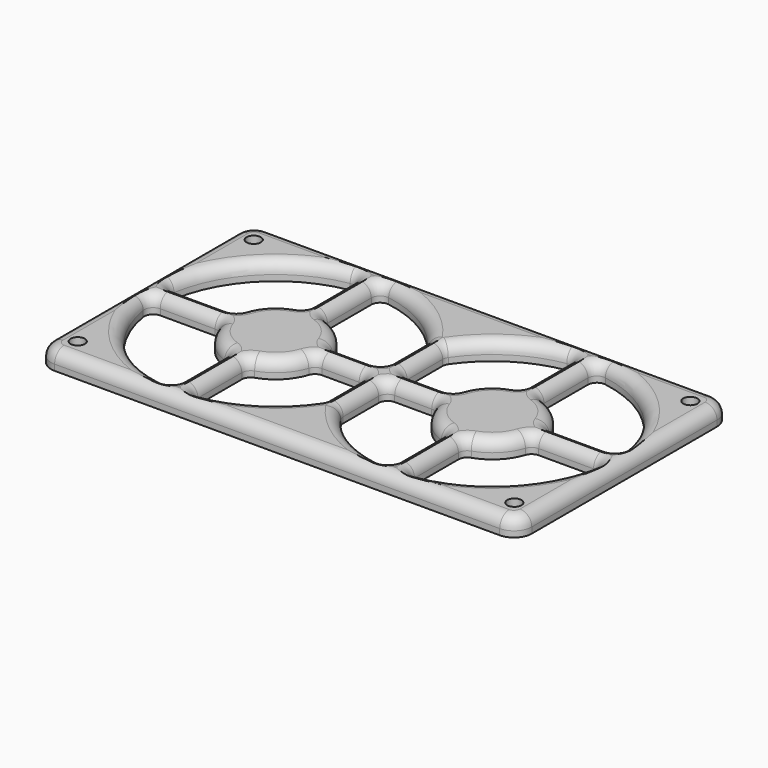
from build123d import *

# Parameters (mm, degrees)
F0_R          = 1.2
F1_DEPTH      = 3
F2_T3_ANGLE   = 71.3351636324
F2_T6_DEPTH   = 9.2412580749
F2_T9_ANGLE   = 53.1830396588
F2_T12_ANGLE  = 53.1830396588
F2_T15_ANGLE  = 46.1876296715
F2_T18_DEPTH  = 7.4731800328
F2_T21_ANGLE  = 53.1830396588
F2_T24_ANGLE  = 53.1830396588
F2_T27_DEPTH  = 39
F2_T30_ANGLE  = 90
F2_T33_ANGLE  = 90
F2_T36_DEPTH  = 75
F2_T39_ANGLE  = 90
F2_T42_DEPTH  = 39
F2_T45_ANGLE  = 90
F2_T48_DEPTH  = 75
F2_T51_ANGLE  = 71.5915198294
F2_T54_ANGLE  = 71.5915198294
F2_T57_DEPTH  = 9.2412580749
F2_T60_ANGLE  = 99.3324181838
F2_T63_ANGLE  = 71.3351636324
F2_T66_ANGLE  = 99.3324181838
F2_T69_DEPTH  = 9.2412580749
F2_T72_ANGLE  = 71.5915198294
F2_T75_ANGLE  = 71.5915198294
F2_T78_DEPTH  = 9.2412580749
F2_T81_ANGLE  = 99.3324181838
F2_T84_ANGLE  = 71.3351636324
F2_T87_ANGLE  = 99.3324181838
F2_T90_DEPTH  = 9.2412580749
F2_T93_ANGLE  = 34.4799521447
F2_T96_ANGLE  = 90
F2_T99_DEPTH  = 6.2361218113
F2_T102_ANGLE = 71.5915198294
F2_T105_ANGLE = 53.1830396588
F2_T108_ANGLE = 71.5915198294
F2_T111_DEPTH = 9.2412580749
F2_T114_ANGLE = 99.3324181838
F2_T117_ANGLE = 46.1876296715
F2_T120_ANGLE = 34.4799521447
F2_T123_ANGLE = 99.3324181838
F2_T126_DEPTH = 9.2412580749
F2_T129_ANGLE = 71.5915198294
F2_T132_ANGLE = 53.1830396588
F2_T135_ANGLE = 71.5915198294
F2_T138_DEPTH = 6.2361218113
F2_T141_ANGLE = 90
F2_T144_DEPTH = 7.4731800328
F2_T147_ANGLE = 71.5915198294
F2_T150_ANGLE = 71.5915198294
F2_T153_DEPTH = 9.2412580749
F2_T156_ANGLE = 99.3324181838
F2_T159_ANGLE = 71.3351636324
F2_T162_ANGLE = 99.3324181838
F2_T165_DEPTH = 9.2412580749
F2_T168_ANGLE = 71.5915198294
F2_T171_ANGLE = 71.5915198294
F2_T174_DEPTH = 9.2412580749
F2_T177_ANGLE = 99.3324181838
F2_T180_ANGLE = 46.1876296715
F2_T183_ANGLE = 34.4799521447
F2_T186_DEPTH = 7.4731800328
F2_T189_ANGLE = 90
F2_T192_DEPTH = 6.2361218113
F2_T195_ANGLE = 99.3324181838
F2_T198_ANGLE = 71.5915198294
F2_T201_ANGLE = 53.1830396588
F2_T204_ANGLE = 71.5915198294
F2_T207_DEPTH = 6.2361218113
F2_T210_ANGLE = 90
F2_T213_DEPTH = 7.4731800328
F2_T216_ANGLE = 34.4799521447
F2_T219_ANGLE = 46.1876296715
F2_T222_ANGLE = 99.3324181838
F2_T225_ANGLE = 99.3324181838
F2_T228_DEPTH = 9.2412580749
F2_T231_ANGLE = 71.5915198294
F2_T234_ANGLE = 53.1830396588
F2_T237_ANGLE = 71.5915198294
F2_T240_DEPTH = 9.2412580749


# Not quite as in the source:
# - a fillet or chamfer that OpenCascade refuses, or shapes differently, is made with other operations: its cross-section is extruded or revolved along the edge and cut away or added


with BuildPart() as f1:
    # F0 (on Top) → F1 (new body)
    with BuildSketch(Plane.XY):
        with BuildLine():
            Line((24.3177403985, -7.9360755384), (-50.6822596015, -7.9360755384))
            ThreePointArc((-50.6822596015, -7.9360755384), (-52.8035799451, -8.8147551948), (-53.6822596015, -10.9360755384))
            Line((-53.6822596015, -10.9360755384), (-53.6822596015, -49.9360755384))
            ThreePointArc((-53.6822596015, -49.9360755384), (-52.8035799451, -52.057395882), (-50.6822596015, -52.9360755384))
            Line((-50.6822596015, -52.9360755384), (24.3177403985, -52.9360755384))
            ThreePointArc((24.3177403985, -52.9360755384), (26.439060742, -52.057395882), (27.3177403985, -49.9360755384))
            Line((27.3177403985, -49.9360755384), (27.3177403985, -10.9360755384))
            ThreePointArc((27.3177403985, -10.9360755384), (26.439060742, -8.8147551948), (24.3177403985, -7.9360755384))
        make_face()
        with Locations((-49.962405785, -48.9713579855)):
            Circle(F0_R, mode=Mode.SUBTRACT)
        with BuildLine():
            ThreePointArc((-34.6703665812, -50.1713579855), (-45.5692589617, -44.5782111621), (-51.162405785, -33.6793187816))
            ThreePointArc((-51.162405785, -33.6793187816), (-50.8256897185, -32.465216348), (-49.6822596015, -31.9360755384))
            Line((-49.6822596015, -31.9360755384), (-40.4410015266, -31.9360755384))
            ThreePointArc((-40.4410015266, -31.9360755384), (-39.5636550488, -32.2194148799), (-39.0177576021, -32.9623913279))
            ThreePointArc((-39.0177576021, -32.9623913279), (-37.0839775875, -36.0929297879), (-33.9534391275, -38.0267098025))
            ThreePointArc((-33.9534391275, -38.0267098025), (-33.2104626795, -38.5726072493), (-32.927123338, -39.4499537271))
            Line((-32.927123338, -39.4499537271), (-32.927123338, -48.6912118019))
            ThreePointArc((-32.927123338, -48.6912118019), (-33.4562641476, -49.8346419189), (-34.6703665812, -50.1713579855))
        make_face(mode=Mode.SUBTRACT)
        with BuildLine():
            ThreePointArc((-28.1838800947, -50.1713579855), (-29.3979825284, -49.8346419189), (-29.927123338, -48.6912118019))
            Line((-29.927123338, -48.6912118019), (-29.927123338, -39.4499537271))
            ThreePointArc((-29.927123338, -39.4499537271), (-29.6437839965, -38.5726072493), (-28.9008075485, -38.0267098025))
            ThreePointArc((-28.9008075485, -38.0267098025), (-25.7702690885, -36.0929297879), (-23.8364890738, -32.9623913279))
            ThreePointArc((-23.8364890738, -32.9623913279), (-23.2905916271, -32.2194148799), (-22.4132451493, -31.9360755384))
            Line((-22.4132451493, -31.9360755384), (-16.177123338, -31.9360755384))
            ThreePointArc((-16.177123338, -31.9360755384), (-15.1164631662, -32.3754153666), (-14.677123338, -33.4360755384))
            Line((-14.677123338, -33.4360755384), (-14.677123338, -40.9092555712))
            ThreePointArc((-14.677123338, -40.9092555712), (-14.7445156231, -41.353817305), (-14.9406368515, -41.7584323306))
            ThreePointArc((-14.9406368515, -41.7584323306), (-20.7028570078, -47.3177256852), (-28.1838800947, -50.1713579855))
        make_face(mode=Mode.SUBTRACT)
        with Locations((23.6081591091, -48.9713579855)):
            Circle(F0_R, mode=Mode.SUBTRACT)
        with BuildLine():
            ThreePointArc((1.8296334188, -50.1713579855), (-5.6513896682, -47.3177256852), (-11.4136098245, -41.7584323306))
            ThreePointArc((-11.4136098245, -41.7584323306), (-11.6097310529, -41.353817305), (-11.677123338, -40.9092555712))
            Line((-11.677123338, -40.9092555712), (-11.677123338, -33.4360755384))
            ThreePointArc((-11.677123338, -33.4360755384), (-11.2377835098, -32.3754153666), (-10.177123338, -31.9360755384))
            Line((-10.177123338, -31.9360755384), (-3.9410015266, -31.9360755384))
            ThreePointArc((-3.9410015266, -31.9360755384), (-3.0636550488, -32.2194148799), (-2.5177576021, -32.9623913279))
            ThreePointArc((-2.5177576021, -32.9623913279), (-0.5839775875, -36.0929297879), (2.5465608725, -38.0267098025))
            ThreePointArc((2.5465608725, -38.0267098025), (3.2895373205, -38.5726072493), (3.572876662, -39.4499537271))
            Line((3.572876662, -39.4499537271), (3.572876662, -48.6912118019))
            ThreePointArc((3.572876662, -48.6912118019), (3.0437358524, -49.8346419189), (1.8296334188, -50.1713579855))
        make_face(mode=Mode.SUBTRACT)
        with BuildLine():
            ThreePointArc((6.572876662, -39.4499537271), (6.8562160035, -38.5726072493), (7.5991924515, -38.0267098025))
            ThreePointArc((7.5991924515, -38.0267098025), (10.7297309115, -36.0929297879), (12.6635109262, -32.9623913279))
            ThreePointArc((12.6635109262, -32.9623913279), (13.2094083729, -32.2194148799), (14.0867548507, -31.9360755384))
            Line((14.0867548507, -31.9360755384), (23.3280129255, -31.9360755384))
            ThreePointArc((23.3280129255, -31.9360755384), (24.4714430425, -32.465216348), (24.8081591091, -33.6793187816))
            ThreePointArc((24.8081591091, -33.6793187816), (19.2150122857, -44.5782111621), (8.3161199053, -50.1713579855))
            ThreePointArc((8.3161199053, -50.1713579855), (7.1020174716, -49.8346419189), (6.572876662, -48.6912118019))
            Line((6.572876662, -48.6912118019), (6.572876662, -39.4499537271))
        make_face(mode=Mode.SUBTRACT)
        with BuildLine():
            ThreePointArc((-34.6703665812, -10.7007930913), (-33.4562641476, -11.0375091579), (-32.927123338, -12.1809392749))
            Line((-32.927123338, -12.1809392749), (-32.927123338, -21.4221973497))
            ThreePointArc((-32.927123338, -21.4221973497), (-33.2104626795, -22.2995438275), (-33.9534391275, -22.8454412743))
            ThreePointArc((-33.9534391275, -22.8454412743), (-37.0839775875, -24.7792212889), (-39.0177576021, -27.9097597489))
            ThreePointArc((-39.0177576021, -27.9097597489), (-39.5636550488, -28.6527361969), (-40.4410015266, -28.9360755384))
            Line((-40.4410015266, -28.9360755384), (-49.6822596015, -28.9360755384))
            ThreePointArc((-49.6822596015, -28.9360755384), (-50.8256897185, -28.4069347288), (-51.162405785, -27.1928322952))
            ThreePointArc((-51.162405785, -27.1928322952), (-45.5692589617, -16.2939399147), (-34.6703665812, -10.7007930913))
        make_face(mode=Mode.SUBTRACT)
        with BuildLine():
            ThreePointArc((-28.9008075485, -22.8454412743), (-29.6437839965, -22.2995438275), (-29.927123338, -21.4221973497))
            Line((-29.927123338, -21.4221973497), (-29.927123338, -12.1809392749))
            ThreePointArc((-29.927123338, -12.1809392749), (-29.3979825284, -11.0375091579), (-28.1838800947, -10.7007930913))
            ThreePointArc((-28.1838800947, -10.7007930913), (-20.7028570078, -13.5544253916), (-14.9406368515, -19.1137187462))
            ThreePointArc((-14.9406368515, -19.1137187462), (-14.7445156231, -19.5183337718), (-14.677123338, -19.9628955056))
            Line((-14.677123338, -19.9628955056), (-14.677123338, -27.4360755384))
            ThreePointArc((-14.677123338, -27.4360755384), (-15.1164631662, -28.4967357102), (-16.177123338, -28.9360755384))
            Line((-16.177123338, -28.9360755384), (-22.4132451493, -28.9360755384))
            ThreePointArc((-22.4132451493, -28.9360755384), (-23.2905916271, -28.6527361969), (-23.8364890738, -27.9097597489))
            ThreePointArc((-23.8364890738, -27.9097597489), (-25.7702690885, -24.7792212889), (-28.9008075485, -22.8454412743))
        make_face(mode=Mode.SUBTRACT)
        with Locations((-49.962405785, -11.9007930913)):
            Circle(F0_R, mode=Mode.SUBTRACT)
        with BuildLine():
            ThreePointArc((1.8296334188, -10.7007930913), (3.0437358524, -11.0375091579), (3.572876662, -12.1809392749))
            Line((3.572876662, -12.1809392749), (3.572876662, -21.4221973497))
            ThreePointArc((3.572876662, -21.4221973497), (3.2895373205, -22.2995438275), (2.5465608725, -22.8454412743))
            ThreePointArc((2.5465608725, -22.8454412743), (-0.5839775875, -24.7792212889), (-2.5177576021, -27.9097597489))
            ThreePointArc((-2.5177576021, -27.9097597489), (-3.0636550488, -28.6527361969), (-3.9410015266, -28.9360755384))
            Line((-3.9410015266, -28.9360755384), (-10.177123338, -28.9360755384))
            ThreePointArc((-10.177123338, -28.9360755384), (-11.2377835098, -28.4967357102), (-11.677123338, -27.4360755384))
            Line((-11.677123338, -27.4360755384), (-11.677123338, -19.9628955056))
            ThreePointArc((-11.677123338, -19.9628955056), (-11.6097310529, -19.5183337718), (-11.4136098245, -19.1137187462))
            ThreePointArc((-11.4136098245, -19.1137187462), (-5.6513896682, -13.5544253916), (1.8296334188, -10.7007930913))
        make_face(mode=Mode.SUBTRACT)
        with BuildLine():
            ThreePointArc((8.3161199053, -10.7007930913), (19.2150122857, -16.2939399147), (24.8081591091, -27.1928322952))
            ThreePointArc((24.8081591091, -27.1928322952), (24.4714430425, -28.4069347288), (23.3280129255, -28.9360755384))
            Line((23.3280129255, -28.9360755384), (14.0867548507, -28.9360755384))
            ThreePointArc((14.0867548507, -28.9360755384), (13.2094083729, -28.6527361969), (12.6635109262, -27.9097597489))
            ThreePointArc((12.6635109262, -27.9097597489), (10.7297309115, -24.7792212889), (7.5991924515, -22.8454412743))
            ThreePointArc((7.5991924515, -22.8454412743), (6.8562160035, -22.2995438275), (6.572876662, -21.4221973497))
            Line((6.572876662, -21.4221973497), (6.572876662, -12.1809392749))
            ThreePointArc((6.572876662, -12.1809392749), (7.1020174716, -11.0375091579), (8.3161199053, -10.7007930913))
        make_face(mode=Mode.SUBTRACT)
        with Locations((23.6081591091, -11.9007930913)):
            Circle(F0_R, mode=Mode.SUBTRACT)
    extrude(amount=F1_DEPTH)

    # F2: fillet of radius 2 on 9 edges, made by hand


with BuildPart() as f2_tool1:
    # F2_s2 → F2_t3 (revolve)
    with BuildSketch(Plane(origin=(9.8097305083, -1.6121047304, 0), x_dir=(0, 0, 1), z_dir=(-0.9867641224, 0.1621621622, 0))):
        with BuildLine():
            ThreePointArc((1, -9.2105987186), (2.4142135624, -8.624812281), (3, -7.2105987186))
            Line((3, -7.2105987186), (3, -9.2105987186))
            Line((3, -9.2105987186), (1, -9.2105987186))
        make_face()
    revolve(axis=Axis((5.072876662, -30.4360755384, 3), (0, 0, -1)), revolution_arc=F2_T3_ANGLE)


with BuildPart() as f2_tool4:
    # F2_s5 → F2_t6 (new body)
    with BuildSketch(Plane.XZ.offset(12.1809392749)):
        with BuildLine():
            ThreePointArc((3.572876662, 1), (4.1586630996, 2.4142135624), (5.572876662, 3))
            Line((5.572876662, 3), (3.572876662, 3))
            Line((3.572876662, 3), (3.572876662, 1))
        make_face()
    extrude(amount=F2_T6_DEPTH)


with BuildPart() as f2_tool7:
    # F2_s8 → F2_t9 (revolve)
    with BuildSketch(Plane(origin=(9.6254528786, -28.920886586, 0), x_dir=(0, 0, 1), z_dir=(-0.3157894737, 0.948829283, 0))):
        with BuildLine():
            ThreePointArc((1, -12.7980983492), (2.4142135624, -12.2123119116), (3, -10.7980983492))
            Line((3, -10.7980983492), (3, -12.7980983492))
            Line((3, -12.7980983492), (1, -12.7980983492))
        make_face()
    revolve(axis=Axis((5.072876662, -30.4360755384, 3), (0, 0, 1)), revolution_arc=F2_T9_ANGLE)


with BuildPart() as f2_tool10:
    # F2_s11 → F2_t12 (revolve)
    with BuildSketch(Plane(origin=(-4.5525762165, -1.5151889524, 0), x_dir=(0, 0, 1), z_dir=(-0.948829283, -0.3157894737, 0))):
        with BuildLine():
            ThreePointArc((1, -38.4806007821), (2.4142135624, -37.8948143445), (3, -36.4806007821))
            Line((3, -36.4806007821), (3, -38.4806007821))
            Line((3, -38.4806007821), (1, -38.4806007821))
        make_face()
    revolve(axis=Axis((5.072876662, -30.4360755384, 3), (0, 0, 1)), revolution_arc=F2_T12_ANGLE)


with BuildPart() as f2_tool13:
    # F2_s14 → F2_t15 (revolve)
    with BuildSketch(Plane(origin=(-24.2755023956, -35.3475649585, 0), x_dir=(0, 0, 1), z_dir=(0.5661178396, 0.8243243243, 0))):
        with BuildLine():
            ThreePointArc((1, 11.324263119), (2.4142135624, 11.9100495567), (3, 13.324263119))
            Line((3, 13.324263119), (3, 11.324263119))
            Line((3, 11.324263119), (1, 11.324263119))
        make_face()
    revolve(axis=Axis((-31.427123338, -30.4360755384, 3), (0, 0, -1)), revolution_arc=F2_T15_ANGLE)


with BuildPart() as f2_tool16:
    # F2_s17 → F2_t18 (new body)
    with BuildSketch(Plane.XZ.offset(19.9628955056)):
        with BuildLine():
            ThreePointArc((-14.677123338, 1), (-14.0913369004, 2.4142135624), (-12.677123338, 3))
            Line((-12.677123338, 3), (-14.677123338, 3))
            Line((-14.677123338, 3), (-14.677123338, 1))
        make_face()
    extrude(amount=F2_T18_DEPTH)


with BuildPart() as f2_tool19:
    # F2_s20 → F2_t21 (revolve)
    with BuildSketch(Plane(origin=(-37.4126870199, -12.4516948987, 0), x_dir=(0, 0, 1), z_dir=(0.948829283, 0.3157894737, 0))):
        with BuildLine():
            ThreePointArc((1, 10.9542849926), (2.4142135624, 11.5400714303), (3, 12.9542849926))
            Line((3, 12.9542849926), (3, 10.9542849926))
            Line((3, 10.9542849926), (1, 10.9542849926))
        make_face()
    revolve(axis=Axis((-31.427123338, -30.4360755384, 3), (0, 0, 1)), revolution_arc=F2_T21_ANGLE)


with BuildPart() as f2_tool22:
    # F2_s23 → F2_t24 (revolve)
    with BuildSketch(Plane(origin=(5.9855636819, -17.9843806397, 0), x_dir=(0, 0, 1), z_dir=(-0.3157894737, 0.948829283, 0))):
        with BuildLine():
            ThreePointArc((1, -47.4303671793), (2.4142135624, -46.8445807417), (3, -45.4303671793))
            Line((3, -45.4303671793), (3, -47.4303671793))
            Line((3, -47.4303671793), (1, -47.4303671793))
        make_face()
    revolve(axis=Axis((-31.427123338, -30.4360755384, 3), (0, 0, 1)), revolution_arc=F2_T24_ANGLE)


with BuildPart() as f2_tool25:
    # F2_s26 → F2_t27 (new body)
    with BuildSketch(Plane.XZ.offset(10.9360755384)):
        with BuildLine():
            ThreePointArc((-53.6822596015, 1), (-53.0964731639, 2.4142135624), (-51.6822596015, 3))
            Line((-51.6822596015, 3), (-53.6822596015, 3))
            Line((-53.6822596015, 3), (-53.6822596015, 1))
        make_face()
    extrude(amount=F2_T27_DEPTH)


with BuildPart() as f2_tool28:
    # F2_s29 → F2_t30 (revolve)
    with BuildSketch(Plane.YZ.offset(-50.6822596015)):
        with BuildLine():
            ThreePointArc((-7.9360755384, 1), (-8.521861976, 2.4142135624), (-9.9360755384, 3))
            Line((-9.9360755384, 3), (-7.9360755384, 3))
            Line((-7.9360755384, 3), (-7.9360755384, 1))
        make_face()
    revolve(axis=Axis((-50.6822596015, -10.9360755384, 3), (0, 0, 1)), revolution_arc=F2_T30_ANGLE)


with BuildPart() as f2_tool31:
    # F2_s32 → F2_t33 (revolve)
    with BuildSketch(Plane.XZ.offset(49.9360755384)):
        with BuildLine():
            ThreePointArc((-53.6822596015, 1), (-53.0964731639, 2.4142135624), (-51.6822596015, 3))
            Line((-51.6822596015, 3), (-53.6822596015, 3))
            Line((-53.6822596015, 3), (-53.6822596015, 1))
        make_face()
    revolve(axis=Axis((-50.6822596015, -49.9360755384, 3), (0, 0, 1)), revolution_arc=F2_T33_ANGLE)


with BuildPart() as f2_tool34:
    # F2_s35 → F2_t36 (new body)
    with BuildSketch(Plane.YZ.offset(-50.6822596015)):
        with BuildLine():
            ThreePointArc((-52.9360755384, 1), (-52.3502891008, 2.4142135624), (-50.9360755384, 3))
            Line((-50.9360755384, 3), (-52.9360755384, 3))
            Line((-52.9360755384, 3), (-52.9360755384, 1))
        make_face()
    extrude(amount=F2_T36_DEPTH)


with BuildPart() as f2_tool37:
    # F2_s38 → F2_t39 (revolve)
    with BuildSketch(Plane.YZ.offset(24.3177403985)):
        with BuildLine():
            ThreePointArc((-52.9360755384, 1), (-52.3502891008, 2.4142135624), (-50.9360755384, 3))
            Line((-50.9360755384, 3), (-52.9360755384, 3))
            Line((-52.9360755384, 3), (-52.9360755384, 1))
        make_face()
    revolve(axis=Axis((24.3177403985, -49.9360755384, 3), (0, 0, 1)), revolution_arc=F2_T39_ANGLE)


with BuildPart() as f2_tool40:
    # F2_s41 → F2_t42 (new body)
    with BuildSketch(Plane.XZ.offset(49.9360755384)):
        with BuildLine():
            ThreePointArc((27.3177403985, 1), (26.7319539609, 2.4142135624), (25.3177403985, 3))
            Line((25.3177403985, 3), (27.3177403985, 3))
            Line((27.3177403985, 3), (27.3177403985, 1))
        make_face()
    extrude(amount=-F2_T42_DEPTH)


with BuildPart() as f2_tool43:
    # F2_s44 → F2_t45 (revolve)
    with BuildSketch(Plane.XZ.offset(10.9360755384)):
        with BuildLine():
            ThreePointArc((27.3177403985, 1), (26.7319539609, 2.4142135624), (25.3177403985, 3))
            Line((25.3177403985, 3), (27.3177403985, 3))
            Line((27.3177403985, 3), (27.3177403985, 1))
        make_face()
    revolve(axis=Axis((24.3177403985, -10.9360755384, 3), (0, 0, 1)), revolution_arc=F2_T45_ANGLE)


with BuildPart() as f2_tool46:
    # F2_s47 → F2_t48 (new body)
    with BuildSketch(Plane.YZ.offset(24.3177403985)):
        with BuildLine():
            ThreePointArc((-7.9360755384, 1), (-8.521861976, 2.4142135624), (-9.9360755384, 3))
            Line((-9.9360755384, 3), (-7.9360755384, 3))
            Line((-7.9360755384, 3), (-7.9360755384, 1))
        make_face()
    extrude(amount=-F2_T48_DEPTH)


with BuildPart() as f2_tool49:
    # F2_s50 → F2_t51 (revolve)
    with BuildSketch(Plane.YZ.offset(-40.4410015266)):
        with BuildLine():
            ThreePointArc((-31.9360755384, 1), (-31.3502891008, 2.4142135624), (-29.9360755384, 3))
            Line((-29.9360755384, 3), (-31.9360755384, 3))
            Line((-31.9360755384, 3), (-31.9360755384, 1))
        make_face()
    revolve(axis=Axis((-40.4410015266, -33.4360755384, 3), (0, 0, -1)), revolution_arc=F2_T51_ANGLE)


with BuildPart() as f2_tool52:
    # F2_s53 → F2_t54 (revolve)
    with BuildSketch(Plane(origin=(-19.1735461372, 6.3813418828, 0), x_dir=(0, 0, 1), z_dir=(-0.948829283, 0.3157894737, 0))):
        with BuildLine():
            ThreePointArc((1, -46.8029944693), (2.4142135624, -46.2172080316), (3, -44.8029944693))
            Line((3, -44.8029944693), (3, -46.8029944693))
            Line((3, -46.8029944693), (1, -46.8029944693))
        make_face()
    revolve(axis=Axis((-34.427123338, -39.4499537271, 3), (0, 0, -1)), revolution_arc=F2_T54_ANGLE)


with BuildPart() as f2_tool55:
    # F2_s56 → F2_t57 (new body)
    with BuildSketch(Plane.XZ.offset(39.4499537271)):
        with BuildLine():
            ThreePointArc((-32.927123338, 1), (-32.3413369004, 2.4142135624), (-30.927123338, 3))
            Line((-30.927123338, 3), (-32.927123338, 3))
            Line((-32.927123338, 3), (-32.927123338, 1))
        make_face()
    extrude(amount=F2_T57_DEPTH)


with BuildPart() as f2_tool58:
    # F2_s59 → F2_t60 (revolve)
    with BuildSketch(Plane.XZ.offset(48.6912118019)):
        with BuildLine():
            ThreePointArc((-32.927123338, 1), (-32.3413369004, 2.4142135624), (-30.927123338, 3))
            Line((-30.927123338, 3), (-32.927123338, 3))
            Line((-32.927123338, 3), (-32.927123338, 1))
        make_face()
    revolve(axis=Axis((-34.427123338, -48.6912118019, 3), (0, 0, -1)), revolution_arc=F2_T60_ANGLE)


with BuildPart() as f2_tool61:
    # F2_s62 → F2_t63 (revolve)
    with BuildSketch(Plane(origin=(-25.7304448022, 4.2284721019, 0), x_dir=(0, 0, 1), z_dir=(0.9867641224, -0.1621621622, 0))):
        with BuildLine():
            ThreePointArc((1, 55.1295176375), (2.4142135624, 55.7153040752), (3, 57.1295176375))
            Line((3, 57.1295176375), (3, 55.1295176375))
            Line((3, 55.1295176375), (1, 55.1295176375))
        make_face()
    revolve(axis=Axis((-31.427123338, -30.4360755384, 3), (0, 0, -1)), revolution_arc=F2_T63_ANGLE)


with BuildPart() as f2_tool64:
    # F2_s65 → F2_t66 (revolve)
    with BuildSketch(Plane(origin=(4.0438276371, -24.6068748472, 0), x_dir=(0, 0, 1), z_dir=(0.1621621622, -0.9867641224, 0))):
        with BuildLine():
            ThreePointArc((1, 55.9467375957), (2.4142135624, 56.5325240333), (3, 57.9467375957))
            Line((3, 57.9467375957), (3, 55.9467375957))
            Line((3, 55.9467375957), (1, 55.9467375957))
        make_face()
    revolve(axis=Axis((-49.6822596015, -33.4360755384, 3), (0, 0, -1)), revolution_arc=F2_T66_ANGLE)


with BuildPart() as f2_tool67:
    # F2_s68 → F2_t69 (new body)
    with BuildSketch(Plane.YZ.offset(-49.6822596015)):
        with BuildLine():
            ThreePointArc((-31.9360755384, 1), (-31.3502891008, 2.4142135624), (-29.9360755384, 3))
            Line((-29.9360755384, 3), (-31.9360755384, 3))
            Line((-31.9360755384, 3), (-31.9360755384, 1))
        make_face()
    extrude(amount=F2_T69_DEPTH)


with BuildPart() as f2_tool70:
    # F2_s71 → F2_t72 (revolve)
    with BuildSketch(Plane.XZ.offset(21.4221973497)):
        with BuildLine():
            ThreePointArc((-32.927123338, 1), (-32.3413369004, 2.4142135624), (-30.927123338, 3))
            Line((-30.927123338, 3), (-32.927123338, 3))
            Line((-32.927123338, 3), (-32.927123338, 1))
        make_face()
    revolve(axis=Axis((-34.427123338, -21.4221973497, 3), (0, 0, -1)), revolution_arc=F2_T72_ANGLE)


with BuildPart() as f2_tool73:
    # F2_s74 → F2_t75 (revolve)
    with BuildSketch(Plane(origin=(-12.2535772008, -36.8174174212, 0), x_dir=(0, 0, 1), z_dir=(0.3157894737, 0.948829283, 0))):
        with BuildLine():
            ThreePointArc((1, -28.2075826288), (2.4142135624, -27.6217961912), (3, -26.2075826288))
            Line((3, -26.2075826288), (3, -28.2075826288))
            Line((3, -28.2075826288), (1, -28.2075826288))
        make_face()
    revolve(axis=Axis((-40.4410015266, -27.4360755384, 3), (0, 0, -1)), revolution_arc=F2_T75_ANGLE)


with BuildPart() as f2_tool76:
    # F2_s77 → F2_t78 (new body)
    with BuildSketch(Plane.YZ.offset(-40.4410015266)):
        with BuildLine():
            ThreePointArc((-28.9360755384, 1), (-29.521861976, 2.4142135624), (-30.9360755384, 3))
            Line((-30.9360755384, 3), (-28.9360755384, 3))
            Line((-28.9360755384, 3), (-28.9360755384, 1))
        make_face()
    extrude(amount=-F2_T78_DEPTH)


with BuildPart() as f2_tool79:
    # F2_s80 → F2_t81 (revolve)
    with BuildSketch(Plane.YZ.offset(-49.6822596015)):
        with BuildLine():
            ThreePointArc((-28.9360755384, 1), (-29.521861976, 2.4142135624), (-30.9360755384, 3))
            Line((-30.9360755384, 3), (-28.9360755384, 3))
            Line((-28.9360755384, 3), (-28.9360755384, 1))
        make_face()
    revolve(axis=Axis((-49.6822596015, -27.4360755384, 3), (0, 0, -1)), revolution_arc=F2_T81_ANGLE)


with BuildPart() as f2_tool82:
    # F2_s83 → F2_t84 (revolve)
    with BuildSketch(Plane(origin=(-5.6966785358, -34.6645476403, 0), x_dir=(0, 0, 1), z_dir=(-0.1621621622, -0.9867641224, 0))):
        with BuildLine():
            ThreePointArc((1, 46.0755779616), (2.4142135624, 46.6613643993), (3, 48.0755779616))
            Line((3, 48.0755779616), (3, 46.0755779616))
            Line((3, 46.0755779616), (1, 46.0755779616))
        make_face()
    revolve(axis=Axis((-31.427123338, -30.4360755384, 3), (0, 0, -1)), revolution_arc=F2_T84_ANGLE)


with BuildPart() as f2_tool85:
    # F2_s86 → F2_t87 (revolve)
    with BuildSketch(Plane(origin=(-35.4709509751, -5.8292006912, 0), x_dir=(0, 0, 1), z_dir=(-0.9867641224, -0.1621621622, 0))):
        with BuildLine():
            ThreePointArc((1, -4.9369370955), (2.4142135624, -4.3511506579), (3, -2.9369370955))
            Line((3, -2.9369370955), (3, -4.9369370955))
            Line((3, -4.9369370955), (1, -4.9369370955))
        make_face()
    revolve(axis=Axis((-34.427123338, -12.1809392749, 3), (0, 0, -1)), revolution_arc=F2_T87_ANGLE)


with BuildPart() as f2_tool88:
    # F2_s89 → F2_t90 (new body)
    with BuildSketch(Plane.XZ.offset(12.1809392749)):
        with BuildLine():
            ThreePointArc((-32.927123338, 1), (-32.3413369004, 2.4142135624), (-30.927123338, 3))
            Line((-30.927123338, 3), (-32.927123338, 3))
            Line((-32.927123338, 3), (-32.927123338, 1))
        make_face()
    extrude(amount=F2_T90_DEPTH)


with BuildPart() as f2_tool91:
    # F2_s92 → F2_t93 (revolve)
    with BuildSketch(Plane(origin=(4.1313820675, -6.0157064361, 0), x_dir=(0, 0, 1), z_dir=(-0.5661178396, 0.8243243243, 0))):
        with BuildLine():
            ThreePointArc((1, -23.1365475411), (2.4142135624, -22.5507611035), (3, -21.1365475411))
            Line((3, -21.1365475411), (3, -23.1365475411))
            Line((3, -23.1365475411), (1, -23.1365475411))
        make_face()
    revolve(axis=Axis((-16.177123338, -19.9628955056, 3), (0, 0, -1)), revolution_arc=F2_T93_ANGLE)


with BuildPart() as f2_tool94:
    # F2_s95 → F2_t96 (revolve)
    with BuildSketch(Plane.XZ.offset(27.4360755384)):
        with BuildLine():
            ThreePointArc((-14.677123338, 1), (-14.0913369004, 2.4142135624), (-12.677123338, 3))
            Line((-12.677123338, 3), (-14.677123338, 3))
            Line((-14.677123338, 3), (-14.677123338, 1))
        make_face()
    revolve(axis=Axis((-16.177123338, -27.4360755384, 3), (0, 0, -1)), revolution_arc=F2_T96_ANGLE)


with BuildPart() as f2_tool97:
    # F2_s98 → F2_t99 (new body)
    with BuildSketch(Plane.YZ.offset(-16.177123338)):
        with BuildLine():
            ThreePointArc((-28.9360755384, 1), (-29.521861976, 2.4142135624), (-30.9360755384, 3))
            Line((-30.9360755384, 3), (-28.9360755384, 3))
            Line((-28.9360755384, 3), (-28.9360755384, 1))
        make_face()
    extrude(amount=-F2_T99_DEPTH)


with BuildPart() as f2_tool100:
    # F2_s101 → F2_t102 (revolve)
    with BuildSketch(Plane.YZ.offset(-22.4132451493)):
        with BuildLine():
            ThreePointArc((-28.9360755384, 1), (-29.521861976, 2.4142135624), (-30.9360755384, 3))
            Line((-30.9360755384, 3), (-28.9360755384, 3))
            Line((-28.9360755384, 3), (-28.9360755384, 1))
        make_face()
    revolve(axis=Axis((-22.4132451493, -27.4360755384, 3), (0, 0, -1)), revolution_arc=F2_T102_ANGLE)


with BuildPart() as f2_tool103:
    # F2_s104 → F2_t105 (revolve)
    with BuildSketch(Plane(origin=(5.9855636819, -17.9843806397, 0), x_dir=(0, 0, 1), z_dir=(0.3157894737, -0.948829283, 0))):
        with BuildLine():
            ThreePointArc((1, 31.4303671793), (2.4142135624, 32.016153617), (3, 33.4303671793))
            Line((3, 33.4303671793), (3, 31.4303671793))
            Line((3, 31.4303671793), (1, 31.4303671793))
        make_face()
    revolve(axis=Axis((-31.427123338, -30.4360755384, 3), (0, 0, 1)), revolution_arc=F2_T105_ANGLE)


with BuildPart() as f2_tool106:
    # F2_s107 → F2_t108 (revolve)
    with BuildSketch(Plane(origin=(-19.1735461372, 6.3813418828, 0), x_dir=(0, 0, 1), z_dir=(0.948829283, -0.3157894737, 0))):
        with BuildLine():
            ThreePointArc((1, 30.8029944693), (2.4142135624, 31.3887809069), (3, 32.8029944693))
            Line((3, 32.8029944693), (3, 30.8029944693))
            Line((3, 30.8029944693), (1, 30.8029944693))
        make_face()
    revolve(axis=Axis((-28.427123338, -21.4221973497, 3), (0, 0, -1)), revolution_arc=F2_T108_ANGLE)


with BuildPart() as f2_tool109:
    # F2_s110 → F2_t111 (new body)
    with BuildSketch(Plane.XZ.offset(21.4221973497)):
        with BuildLine():
            ThreePointArc((-29.927123338, 1), (-30.5129097756, 2.4142135624), (-31.927123338, 3))
            Line((-31.927123338, 3), (-29.927123338, 3))
            Line((-29.927123338, 3), (-29.927123338, 1))
        make_face()
    extrude(amount=-F2_T111_DEPTH)


with BuildPart() as f2_tool112:
    # F2_s113 → F2_t114 (revolve)
    with BuildSketch(Plane.XZ.offset(12.1809392749)):
        with BuildLine():
            ThreePointArc((-29.927123338, 1), (-30.5129097756, 2.4142135624), (-31.927123338, 3))
            Line((-31.927123338, 3), (-29.927123338, 3))
            Line((-29.927123338, 3), (-29.927123338, 1))
        make_face()
    revolve(axis=Axis((-28.427123338, -12.1809392749, 3), (0, 0, -1)), revolution_arc=F2_T114_ANGLE)


with BuildPart() as f2_tool115:
    # F2_s116 → F2_t117 (revolve)
    with BuildSketch(Plane(origin=(-25.7304448022, 4.2284721019, 0), x_dir=(0, 0, 1), z_dir=(-0.9867641224, 0.1621621622, 0))):
        with BuildLine():
            ThreePointArc((1, -15.1295176375), (2.4142135624, -14.5437311999), (3, -13.1295176375))
            Line((3, -13.1295176375), (3, -15.1295176375))
            Line((3, -15.1295176375), (1, -15.1295176375))
        make_face()
    revolve(axis=Axis((-31.427123338, -30.4360755384, 3), (0, 0, -1)), revolution_arc=F2_T117_ANGLE)


with BuildPart() as f2_tool118:
    # F2_s119 → F2_t120 (revolve)
    with BuildSketch(Plane.XZ.offset(40.9092555712)):
        with BuildLine():
            ThreePointArc((-14.677123338, 1), (-14.0913369004, 2.4142135624), (-12.677123338, 3))
            Line((-12.677123338, 3), (-14.677123338, 3))
            Line((-14.677123338, 3), (-14.677123338, 1))
        make_face()
    revolve(axis=Axis((-16.177123338, -40.9092555712, 3), (0, 0, -1)), revolution_arc=F2_T120_ANGLE)


with BuildPart() as f2_tool121:
    # F2_s122 → F2_t123 (revolve)
    with BuildSketch(Plane(origin=(-35.4709509751, -5.8292006912, 0), x_dir=(0, 0, 1), z_dir=(0.9867641224, 0.1621621622, 0))):
        with BuildLine():
            ThreePointArc((1, 44.9369370955), (2.4142135624, 45.5227235331), (3, 46.9369370955))
            Line((3, 46.9369370955), (3, 44.9369370955))
            Line((3, 44.9369370955), (1, 44.9369370955))
        make_face()
    revolve(axis=Axis((-28.427123338, -48.6912118019, 3), (0, 0, -1)), revolution_arc=F2_T123_ANGLE)


with BuildPart() as f2_tool124:
    # F2_s125 → F2_t126 (new body)
    with BuildSketch(Plane.XZ.offset(48.6912118019)):
        with BuildLine():
            ThreePointArc((-29.927123338, 1), (-30.5129097756, 2.4142135624), (-31.927123338, 3))
            Line((-31.927123338, 3), (-29.927123338, 3))
            Line((-29.927123338, 3), (-29.927123338, 1))
        make_face()
    extrude(amount=-F2_T126_DEPTH)


with BuildPart() as f2_tool127:
    # F2_s128 → F2_t129 (revolve)
    with BuildSketch(Plane.XZ.offset(39.4499537271)):
        with BuildLine():
            ThreePointArc((-29.927123338, 1), (-30.5129097756, 2.4142135624), (-31.927123338, 3))
            Line((-31.927123338, 3), (-29.927123338, 3))
            Line((-29.927123338, 3), (-29.927123338, 1))
        make_face()
    revolve(axis=Axis((-28.427123338, -39.4499537271, 3), (0, 0, -1)), revolution_arc=F2_T129_ANGLE)


with BuildPart() as f2_tool130:
    # F2_s131 → F2_t132 (revolve)
    with BuildSketch(Plane(origin=(-37.4126870199, -12.4516948987, 0), x_dir=(0, 0, 1), z_dir=(-0.948829283, -0.3157894737, 0))):
        with BuildLine():
            ThreePointArc((1, -26.9542849926), (2.4142135624, -26.368498555), (3, -24.9542849926))
            Line((3, -24.9542849926), (3, -26.9542849926))
            Line((3, -26.9542849926), (1, -26.9542849926))
        make_face()
    revolve(axis=Axis((-31.427123338, -30.4360755384, 3), (0, 0, 1)), revolution_arc=F2_T132_ANGLE)


with BuildPart() as f2_tool133:
    # F2_s134 → F2_t135 (revolve)
    with BuildSketch(Plane(origin=(-12.2535772008, -36.8174174212, 0), x_dir=(0, 0, 1), z_dir=(-0.3157894737, -0.948829283, 0))):
        with BuildLine():
            ThreePointArc((1, 12.2075826288), (2.4142135624, 12.7933690664), (3, 14.2075826288))
            Line((3, 14.2075826288), (3, 12.2075826288))
            Line((3, 12.2075826288), (1, 12.2075826288))
        make_face()
    revolve(axis=Axis((-22.4132451493, -33.4360755384, 3), (0, 0, -1)), revolution_arc=F2_T135_ANGLE)


with BuildPart() as f2_tool136:
    # F2_s137 → F2_t138 (new body)
    with BuildSketch(Plane.YZ.offset(-22.4132451493)):
        with BuildLine():
            ThreePointArc((-31.9360755384, 1), (-31.3502891008, 2.4142135624), (-29.9360755384, 3))
            Line((-29.9360755384, 3), (-31.9360755384, 3))
            Line((-31.9360755384, 3), (-31.9360755384, 1))
        make_face()
    extrude(amount=F2_T138_DEPTH)


with BuildPart() as f2_tool139:
    # F2_s140 → F2_t141 (revolve)
    with BuildSketch(Plane.YZ.offset(-16.177123338)):
        with BuildLine():
            ThreePointArc((-31.9360755384, 1), (-31.3502891008, 2.4142135624), (-29.9360755384, 3))
            Line((-29.9360755384, 3), (-31.9360755384, 3))
            Line((-31.9360755384, 3), (-31.9360755384, 1))
        make_face()
    revolve(axis=Axis((-16.177123338, -33.4360755384, 3), (0, 0, -1)), revolution_arc=F2_T141_ANGLE)


with BuildPart() as f2_tool142:
    # F2_s143 → F2_t144 (new body)
    with BuildSketch(Plane.XZ.offset(33.4360755384)):
        with BuildLine():
            ThreePointArc((-14.677123338, 1), (-14.0913369004, 2.4142135624), (-12.677123338, 3))
            Line((-12.677123338, 3), (-14.677123338, 3))
            Line((-14.677123338, 3), (-14.677123338, 1))
        make_face()
    extrude(amount=F2_T144_DEPTH)


with BuildPart() as f2_tool145:
    # F2_s146 → F2_t147 (revolve)
    with BuildSketch(Plane.XZ.offset(39.4499537271)):
        with BuildLine():
            ThreePointArc((6.572876662, 1), (5.9870902244, 2.4142135624), (4.572876662, 3))
            Line((4.572876662, 3), (6.572876662, 3))
            Line((6.572876662, 3), (6.572876662, 1))
        make_face()
    revolve(axis=Axis((8.072876662, -39.4499537271, 3), (0, 0, -1)), revolution_arc=F2_T147_ANGLE)


with BuildPart() as f2_tool148:
    # F2_s149 → F2_t150 (revolve)
    with BuildSketch(Plane(origin=(-8.6136880041, -25.8809114748, 0), x_dir=(0, 0, 1), z_dir=(-0.3157894737, -0.948829283, 0))):
        with BuildLine():
            ThreePointArc((1, -22.4246862013), (2.4142135624, -21.8388997637), (3, -20.4246862013))
            Line((3, -20.4246862013), (3, -22.4246862013))
            Line((3, -22.4246862013), (1, -22.4246862013))
        make_face()
    revolve(axis=Axis((14.0867548507, -33.4360755384, 3), (0, 0, -1)), revolution_arc=F2_T150_ANGLE)


with BuildPart() as f2_tool151:
    # F2_s152 → F2_t153 (new body)
    with BuildSketch(Plane.YZ.offset(14.0867548507)):
        with BuildLine():
            ThreePointArc((-31.9360755384, 1), (-31.3502891008, 2.4142135624), (-29.9360755384, 3))
            Line((-29.9360755384, 3), (-31.9360755384, 3))
            Line((-31.9360755384, 3), (-31.9360755384, 1))
        make_face()
    extrude(amount=F2_T153_DEPTH)


with BuildPart() as f2_tool154:
    # F2_s155 → F2_t156 (revolve)
    with BuildSketch(Plane.YZ.offset(23.3280129255)):
        with BuildLine():
            ThreePointArc((-31.9360755384, 1), (-31.3502891008, 2.4142135624), (-29.9360755384, 3))
            Line((-29.9360755384, 3), (-31.9360755384, 3))
            Line((-31.9360755384, 3), (-31.9360755384, 1))
        make_face()
    revolve(axis=Axis((23.3280129255, -33.4360755384, 3), (0, 0, -1)), revolution_arc=F2_T156_ANGLE)


with BuildPart() as f2_tool157:
    # F2_s158 → F2_t159 (revolve)
    with BuildSketch(Plane(origin=(-4.7368538463, -28.823970808, 0), x_dir=(0, 0, 1), z_dir=(0.1621621622, 0.9867641224, 0))):
        with BuildLine():
            ThreePointArc((1, 29.9413125042), (2.4142135624, 30.5270989419), (3, 31.9413125042))
            Line((3, 31.9413125042), (3, 29.9413125042))
            Line((3, 29.9413125042), (1, 29.9413125042))
        make_face()
    revolve(axis=Axis((5.072876662, -30.4360755384, 3), (0, 0, -1)), revolution_arc=F2_T159_ANGLE)


with BuildPart() as f2_tool160:
    # F2_s161 → F2_t162 (revolve)
    with BuildSketch(Plane(origin=(0.0692243354, 0.0113761411, 0), x_dir=(0, 0, 1), z_dir=(0.9867641224, 0.1621621622, 0))):
        with BuildLine():
            ThreePointArc((1, 50.8558560144), (2.4142135624, 51.441642452), (3, 52.8558560144))
            Line((3, 52.8558560144), (3, 50.8558560144))
            Line((3, 50.8558560144), (1, 50.8558560144))
        make_face()
    revolve(axis=Axis((8.072876662, -48.6912118019, 3), (0, 0, -1)), revolution_arc=F2_T162_ANGLE)


with BuildPart() as f2_tool163:
    # F2_s164 → F2_t165 (new body)
    with BuildSketch(Plane.XZ.offset(48.6912118019)):
        with BuildLine():
            ThreePointArc((6.572876662, 1), (5.9870902244, 2.4142135624), (4.572876662, 3))
            Line((4.572876662, 3), (6.572876662, 3))
            Line((6.572876662, 3), (6.572876662, 1))
        make_face()
    extrude(amount=-F2_T165_DEPTH)


with BuildPart() as f2_tool166:
    # F2_s167 → F2_t168 (revolve)
    with BuildSketch(Plane.YZ.offset(-3.9410015266)):
        with BuildLine():
            ThreePointArc((-31.9360755384, 1), (-31.3502891008, 2.4142135624), (-29.9360755384, 3))
            Line((-29.9360755384, 3), (-31.9360755384, 3))
            Line((-31.9360755384, 3), (-31.9360755384, 1))
        make_face()
    revolve(axis=Axis((-3.9410015266, -33.4360755384, 3), (0, 0, -1)), revolution_arc=F2_T168_ANGLE)


with BuildPart() as f2_tool169:
    # F2_s170 → F2_t171 (revolve)
    with BuildSketch(Plane(origin=(13.6865646662, -4.5551640636, 0), x_dir=(0, 0, 1), z_dir=(-0.948829283, 0.3157894737, 0))):
        with BuildLine():
            ThreePointArc((1, -35.2766786798), (2.4142135624, -34.6908922422), (3, -33.2766786798))
            Line((3, -33.2766786798), (3, -35.2766786798))
            Line((3, -35.2766786798), (1, -35.2766786798))
        make_face()
    revolve(axis=Axis((2.072876662, -39.4499537271, 3), (0, 0, -1)), revolution_arc=F2_T171_ANGLE)


with BuildPart() as f2_tool172:
    # F2_s173 → F2_t174 (new body)
    with BuildSketch(Plane.XZ.offset(39.4499537271)):
        with BuildLine():
            ThreePointArc((3.572876662, 1), (4.1586630996, 2.4142135624), (5.572876662, 3))
            Line((5.572876662, 3), (3.572876662, 3))
            Line((3.572876662, 3), (3.572876662, 1))
        make_face()
    extrude(amount=F2_T174_DEPTH)


with BuildPart() as f2_tool175:
    # F2_s176 → F2_t177 (revolve)
    with BuildSketch(Plane.XZ.offset(48.6912118019)):
        with BuildLine():
            ThreePointArc((3.572876662, 1), (4.1586630996, 2.4142135624), (5.572876662, 3))
            Line((5.572876662, 3), (3.572876662, 3))
            Line((3.572876662, 3), (3.572876662, 1))
        make_face()
    revolve(axis=Axis((2.072876662, -48.6912118019, 3), (0, 0, -1)), revolution_arc=F2_T177_ANGLE)


with BuildPart() as f2_tool178:
    # F2_s179 → F2_t180 (revolve)
    with BuildSketch(Plane(origin=(9.8097305083, -1.6121047304, 0), x_dir=(0, 0, 1), z_dir=(0.9867641224, -0.1621621622, 0))):
        with BuildLine():
            ThreePointArc((1, 49.2105987186), (2.4142135624, 49.7963851562), (3, 51.2105987186))
            Line((3, 51.2105987186), (3, 49.2105987186))
            Line((3, 49.2105987186), (1, 49.2105987186))
        make_face()
    revolve(axis=Axis((5.072876662, -30.4360755384, 3), (0, 0, -1)), revolution_arc=F2_T180_ANGLE)


with BuildPart() as f2_tool181:
    # F2_s182 → F2_t183 (revolve)
    with BuildSketch(Plane(origin=(15.8292454715, -23.0489681915, 0), x_dir=(0, 0, 1), z_dir=(0.5661178396, -0.8243243243, 0))):
        with BuildLine():
            ThreePointArc((1, 33.0487097033), (2.4142135624, 33.6344961409), (3, 35.0487097033))
            Line((3, 35.0487097033), (3, 33.0487097033))
            Line((3, 33.0487097033), (1, 33.0487097033))
        make_face()
    revolve(axis=Axis((-10.177123338, -40.9092555712, 3), (0, 0, -1)), revolution_arc=F2_T183_ANGLE)


with BuildPart() as f2_tool184:
    # F2_s185 → F2_t186 (new body)
    with BuildSketch(Plane.XZ.offset(40.9092555712)):
        with BuildLine():
            ThreePointArc((-11.677123338, 1), (-12.2629097756, 2.4142135624), (-13.677123338, 3))
            Line((-13.677123338, 3), (-11.677123338, 3))
            Line((-11.677123338, 3), (-11.677123338, 1))
        make_face()
    extrude(amount=-F2_T186_DEPTH)


with BuildPart() as f2_tool187:
    # F2_s188 → F2_t189 (revolve)
    with BuildSketch(Plane.XZ.offset(33.4360755384)):
        with BuildLine():
            ThreePointArc((-11.677123338, 1), (-12.2629097756, 2.4142135624), (-13.677123338, 3))
            Line((-13.677123338, 3), (-11.677123338, 3))
            Line((-11.677123338, 3), (-11.677123338, 1))
        make_face()
    revolve(axis=Axis((-10.177123338, -33.4360755384, 3), (0, 0, -1)), revolution_arc=F2_T189_ANGLE)


with BuildPart() as f2_tool190:
    # F2_s191 → F2_t192 (new body)
    with BuildSketch(Plane.YZ.offset(-10.177123338)):
        with BuildLine():
            ThreePointArc((-31.9360755384, 1), (-31.3502891008, 2.4142135624), (-29.9360755384, 3))
            Line((-29.9360755384, 3), (-31.9360755384, 3))
            Line((-31.9360755384, 3), (-31.9360755384, 1))
        make_face()
    extrude(amount=F2_T192_DEPTH)


with BuildPart() as f2_tool193:
    # F2_s194 → F2_t195 (revolve)
    with BuildSketch(Plane(origin=(0.0692243354, 0.0113761411, 0), x_dir=(0, 0, 1), z_dir=(-0.9867641224, -0.1621621622, 0))):
        with BuildLine():
            ThreePointArc((1, -10.8558560144), (2.4142135624, -10.2700695768), (3, -8.8558560144))
            Line((3, -8.8558560144), (3, -10.8558560144))
            Line((3, -10.8558560144), (1, -10.8558560144))
        make_face()
    revolve(axis=Axis((2.072876662, -12.1809392749, 3), (0, 0, -1)), revolution_arc=F2_T195_ANGLE)


with BuildPart() as f2_tool196:
    # F2_s197 → F2_t198 (revolve)
    with BuildSketch(Plane.XZ.offset(21.4221973497)):
        with BuildLine():
            ThreePointArc((3.572876662, 1), (4.1586630996, 2.4142135624), (5.572876662, 3))
            Line((5.572876662, 3), (3.572876662, 3))
            Line((3.572876662, 3), (3.572876662, 1))
        make_face()
    revolve(axis=Axis((2.072876662, -21.4221973497, 3), (0, 0, -1)), revolution_arc=F2_T198_ANGLE)


with BuildPart() as f2_tool199:
    # F2_s200 → F2_t201 (revolve)
    with BuildSketch(Plane(origin=(-4.5525762165, -1.5151889524, 0), x_dir=(0, 0, 1), z_dir=(0.948829283, 0.3157894737, 0))):
        with BuildLine():
            ThreePointArc((1, 22.4806007821), (2.4142135624, 23.0663872197), (3, 24.4806007821))
            Line((3, 24.4806007821), (3, 22.4806007821))
            Line((3, 22.4806007821), (1, 22.4806007821))
        make_face()
    revolve(axis=Axis((5.072876662, -30.4360755384, 3), (0, 0, 1)), revolution_arc=F2_T201_ANGLE)


with BuildPart() as f2_tool202:
    # F2_s203 → F2_t204 (revolve)
    with BuildSketch(Plane(origin=(-8.6136880041, -25.8809114748, 0), x_dir=(0, 0, 1), z_dir=(0.3157894737, 0.948829283, 0))):
        with BuildLine():
            ThreePointArc((1, 6.4246862013), (2.4142135624, 7.010472639), (3, 8.4246862013))
            Line((3, 8.4246862013), (3, 6.4246862013))
            Line((3, 6.4246862013), (1, 6.4246862013))
        make_face()
    revolve(axis=Axis((-3.9410015266, -27.4360755384, 3), (0, 0, -1)), revolution_arc=F2_T204_ANGLE)


with BuildPart() as f2_tool205:
    # F2_s206 → F2_t207 (new body)
    with BuildSketch(Plane.YZ.offset(-3.9410015266)):
        with BuildLine():
            ThreePointArc((-28.9360755384, 1), (-29.521861976, 2.4142135624), (-30.9360755384, 3))
            Line((-30.9360755384, 3), (-28.9360755384, 3))
            Line((-28.9360755384, 3), (-28.9360755384, 1))
        make_face()
    extrude(amount=-F2_T207_DEPTH)


with BuildPart() as f2_tool208:
    # F2_s209 → F2_t210 (revolve)
    with BuildSketch(Plane.YZ.offset(-10.177123338)):
        with BuildLine():
            ThreePointArc((-28.9360755384, 1), (-29.521861976, 2.4142135624), (-30.9360755384, 3))
            Line((-30.9360755384, 3), (-28.9360755384, 3))
            Line((-28.9360755384, 3), (-28.9360755384, 1))
        make_face()
    revolve(axis=Axis((-10.177123338, -27.4360755384, 3), (0, 0, -1)), revolution_arc=F2_T210_ANGLE)


with BuildPart() as f2_tool211:
    # F2_s212 → F2_t213 (new body)
    with BuildSketch(Plane.XZ.offset(27.4360755384)):
        with BuildLine():
            ThreePointArc((-11.677123338, 1), (-12.2629097756, 2.4142135624), (-13.677123338, 3))
            Line((-13.677123338, 3), (-11.677123338, 3))
            Line((-11.677123338, 3), (-11.677123338, 1))
        make_face()
    extrude(amount=-F2_T213_DEPTH)


with BuildPart() as f2_tool214:
    # F2_s215 → F2_t216 (revolve)
    with BuildSketch(Plane.XZ.offset(19.9628955056)):
        with BuildLine():
            ThreePointArc((-11.677123338, 1), (-12.2629097756, 2.4142135624), (-13.677123338, 3))
            Line((-13.677123338, 3), (-11.677123338, 3))
            Line((-11.677123338, 3), (-11.677123338, 1))
        make_face()
    revolve(axis=Axis((-10.177123338, -19.9628955056, 3), (0, 0, -1)), revolution_arc=F2_T216_ANGLE)


with BuildPart() as f2_tool217:
    # F2_s218 → F2_t219 (revolve)
    with BuildSketch(Plane(origin=(-12.5776389916, -18.3143032031, 0), x_dir=(0, 0, 1), z_dir=(-0.5661178396, -0.8243243243, 0))):
        with BuildLine():
            ThreePointArc((1, -1.4121009569), (2.4142135624, -0.8263145192), (3, 0.5878990431))
            Line((3, 0.5878990431), (3, -1.4121009569))
            Line((3, -1.4121009569), (1, -1.4121009569))
        make_face()
    revolve(axis=Axis((5.072876662, -30.4360755384, 3), (0, 0, -1)), revolution_arc=F2_T219_ANGLE)


with BuildPart() as f2_tool220:
    # F2_s221 → F2_t222 (revolve)
    with BuildSketch(Plane.XZ.offset(12.1809392749)):
        with BuildLine():
            ThreePointArc((6.572876662, 1), (5.9870902244, 2.4142135624), (4.572876662, 3))
            Line((4.572876662, 3), (6.572876662, 3))
            Line((6.572876662, 3), (6.572876662, 1))
        make_face()
    revolve(axis=Axis((8.072876662, -12.1809392749, 3), (0, 0, -1)), revolution_arc=F2_T222_ANGLE)


with BuildPart() as f2_tool223:
    # F2_s224 → F2_t225 (revolve)
    with BuildSketch(Plane(origin=(5.0036523267, -30.4474516795, 0), x_dir=(0, 0, 1), z_dir=(-0.1621621622, 0.9867641224, 0))):
        with BuildLine():
            ThreePointArc((1, 20.0701528702), (2.4142135624, 20.6559393078), (3, 22.0701528702))
            Line((3, 22.0701528702), (3, 20.0701528702))
            Line((3, 20.0701528702), (1, 20.0701528702))
        make_face()
    revolve(axis=Axis((23.3280129255, -27.4360755384, 3), (0, 0, -1)), revolution_arc=F2_T225_ANGLE)


with BuildPart() as f2_tool226:
    # F2_s227 → F2_t228 (new body)
    with BuildSketch(Plane.YZ.offset(23.3280129255)):
        with BuildLine():
            ThreePointArc((-28.9360755384, 1), (-29.521861976, 2.4142135624), (-30.9360755384, 3))
            Line((-30.9360755384, 3), (-28.9360755384, 3))
            Line((-28.9360755384, 3), (-28.9360755384, 1))
        make_face()
    extrude(amount=-F2_T228_DEPTH)


with BuildPart() as f2_tool229:
    # F2_s230 → F2_t231 (revolve)
    with BuildSketch(Plane.YZ.offset(14.0867548507)):
        with BuildLine():
            ThreePointArc((-28.9360755384, 1), (-29.521861976, 2.4142135624), (-30.9360755384, 3))
            Line((-30.9360755384, 3), (-28.9360755384, 3))
            Line((-28.9360755384, 3), (-28.9360755384, 1))
        make_face()
    revolve(axis=Axis((14.0867548507, -27.4360755384, 3), (0, 0, -1)), revolution_arc=F2_T231_ANGLE)


with BuildPart() as f2_tool232:
    # F2_s233 → F2_t234 (revolve)
    with BuildSketch(Plane(origin=(9.6254528786, -28.920886586, 0), x_dir=(0, 0, 1), z_dir=(0.3157894737, -0.948829283, 0))):
        with BuildLine():
            ThreePointArc((1, -3.2019016508), (2.4142135624, -2.6161152131), (3, -1.2019016508))
            Line((3, -1.2019016508), (3, -3.2019016508))
            Line((3, -3.2019016508), (1, -3.2019016508))
        make_face()
    revolve(axis=Axis((5.072876662, -30.4360755384, 3), (0, 0, 1)), revolution_arc=F2_T234_ANGLE)


with BuildPart() as f2_tool235:
    # F2_s236 → F2_t237 (revolve)
    with BuildSketch(Plane(origin=(13.6865646662, -4.5551640636, 0), x_dir=(0, 0, 1), z_dir=(0.948829283, -0.3157894737, 0))):
        with BuildLine():
            ThreePointArc((1, 19.2766786798), (2.4142135624, 19.8624651174), (3, 21.2766786798))
            Line((3, 21.2766786798), (3, 19.2766786798))
            Line((3, 19.2766786798), (1, 19.2766786798))
        make_face()
    revolve(axis=Axis((8.072876662, -21.4221973497, 3), (0, 0, -1)), revolution_arc=F2_T237_ANGLE)


with BuildPart() as f2_tool238:
    # F2_s239 → F2_t240 (new body)
    with BuildSketch(Plane.XZ.offset(21.4221973497)):
        with BuildLine():
            ThreePointArc((6.572876662, 1), (5.9870902244, 2.4142135624), (4.572876662, 3))
            Line((4.572876662, 3), (6.572876662, 3))
            Line((6.572876662, 3), (6.572876662, 1))
        make_face()
    extrude(amount=-F2_T240_DEPTH)


with BuildPart() as f1_1:
    add(f1.part)

    # F2_t241: cut F2_tool1, F2_tool4, F2_tool7, F2_tool10, F2_tool13, F2_tool16, F2_tool19, F2_tool22, F2_tool25, F2_tool28, F2_tool31, F2_tool34, F2_tool37, F2_tool40, F2_tool43, F2_tool46, F2_tool49, F2_tool52, F2_tool55, F2_tool58, F2_tool61, F2_tool64, F2_tool67, F2_tool70, F2_tool73, F2_tool76, F2_tool79, F2_tool82, F2_tool85, F2_tool88, F2_tool91, F2_tool94, F2_tool97, F2_tool100, F2_tool103, F2_tool106, F2_tool109, F2_tool112, F2_tool115, F2_tool118, F2_tool121, F2_tool124, F2_tool127, F2_tool130, F2_tool133, F2_tool136, F2_tool139, F2_tool142, F2_tool145, F2_tool148, F2_tool151, F2_tool154, F2_tool157, F2_tool160, F2_tool163, F2_tool166, F2_tool169, F2_tool172, F2_tool175, F2_tool178, F2_tool181, F2_tool184, F2_tool187, F2_tool190, F2_tool193, F2_tool196, F2_tool199, F2_tool202, F2_tool205, F2_tool208, F2_tool211, F2_tool214, F2_tool217, F2_tool220, F2_tool223, F2_tool226, F2_tool229, F2_tool232, F2_tool235, F2_tool238
    add([f2_tool1.part, f2_tool4.part, f2_tool7.part, f2_tool10.part, f2_tool13.part, f2_tool16.part, f2_tool19.part, f2_tool22.part, f2_tool25.part, f2_tool28.part, f2_tool31.part, f2_tool34.part, f2_tool37.part, f2_tool40.part, f2_tool43.part, f2_tool46.part, f2_tool49.part, f2_tool52.part, f2_tool55.part, f2_tool58.part, f2_tool61.part, f2_tool64.part, f2_tool67.part, f2_tool70.part, f2_tool73.part, f2_tool76.part, f2_tool79.part, f2_tool82.part, f2_tool85.part, f2_tool88.part, f2_tool91.part, f2_tool94.part, f2_tool97.part, f2_tool100.part, f2_tool103.part, f2_tool106.part, f2_tool109.part, f2_tool112.part, f2_tool115.part, f2_tool118.part, f2_tool121.part, f2_tool124.part, f2_tool127.part, f2_tool130.part, f2_tool133.part, f2_tool136.part, f2_tool139.part, f2_tool142.part, f2_tool145.part, f2_tool148.part, f2_tool151.part, f2_tool154.part, f2_tool157.part, f2_tool160.part, f2_tool163.part, f2_tool166.part, f2_tool169.part, f2_tool172.part, f2_tool175.part, f2_tool178.part, f2_tool181.part, f2_tool184.part, f2_tool187.part, f2_tool190.part, f2_tool193.part, f2_tool196.part, f2_tool199.part, f2_tool202.part, f2_tool205.part, f2_tool208.part, f2_tool211.part, f2_tool214.part, f2_tool217.part, f2_tool220.part, f2_tool223.part, f2_tool226.part, f2_tool229.part, f2_tool232.part, f2_tool235.part, f2_tool238.part], mode=Mode.SUBTRACT)


solid = f1_1.part
